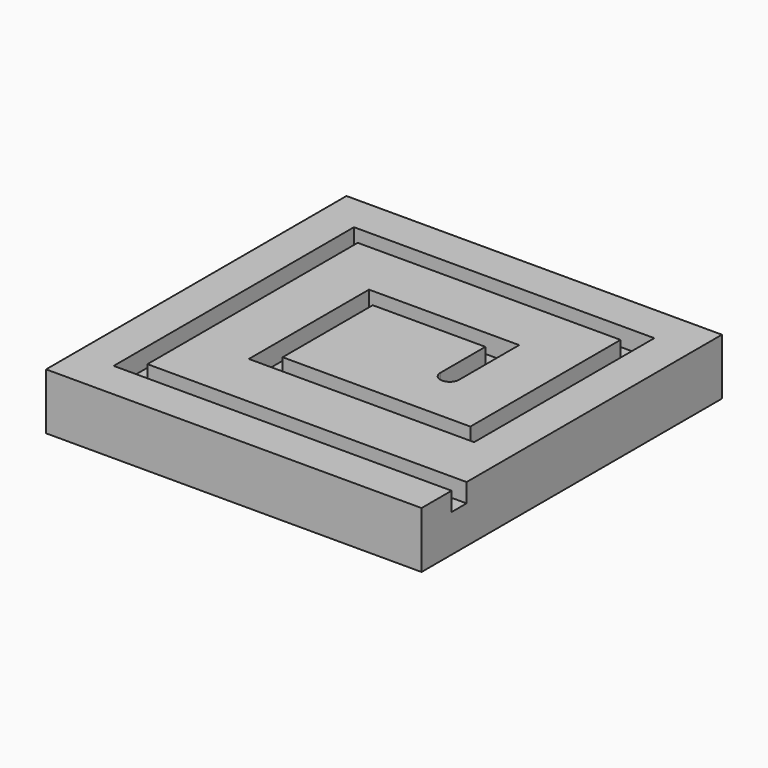
from build123d import *

# Parameters (mm, degrees)
F0_W     = 100
F0_H     = 100
F1_DEPTH = 15
F3_DEPTH = 5
F4_R     = 2.5
F5_DEPTH = 15.001


with BuildPart() as f1:
    # F0 (on Top) → F1 (new body)
    with BuildSketch(Plane.XY):
        Rectangle(F0_W, F0_H)
    extrude(amount=F1_DEPTH)

    # F2 (on face) → F3 (cut)
    with BuildSketch(Plane.XY.offset(15)):
        Polygon((-40, -40), (50, -40), (50, -35), (-35, -35), (-35, 35), (35, 35), (35, -15), (-15, -15), (-15, 15), (15, 15), (15, 0), (20, 0), (20, 20), (-20, 20), (-20, -20), (40, -20), (40, 40), (-40, 40), align=None)
    extrude(amount=-F3_DEPTH, mode=Mode.SUBTRACT)

    # F4 (on face) → F5 (cut, through all)
    with BuildSketch(Plane.XY.offset(15)):
        with Locations((17.5, 0)):
            Circle(F4_R)
    extrude(amount=-F5_DEPTH, mode=Mode.SUBTRACT)


solid = f1.part
